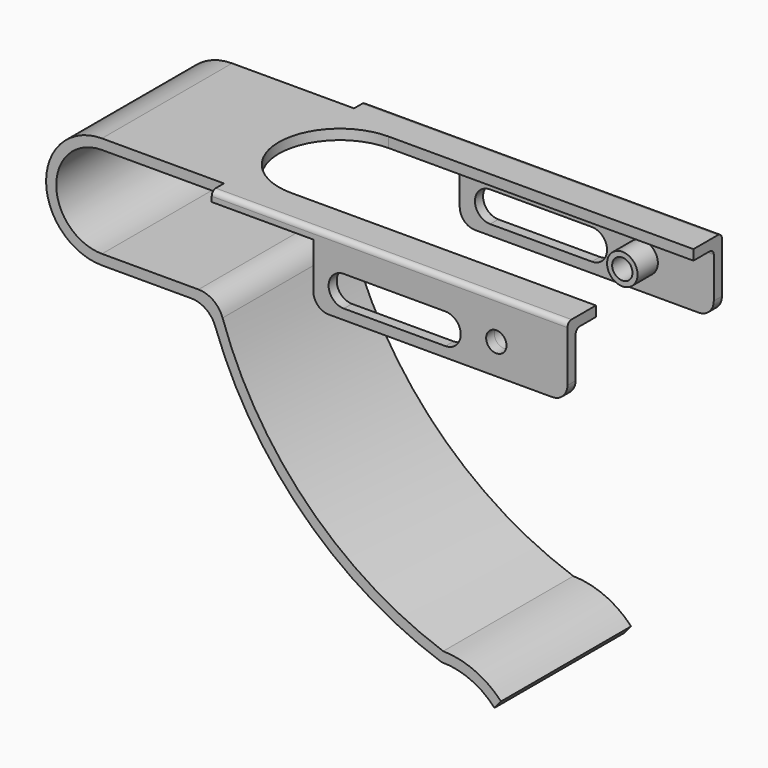
from build123d import *

# Parameters (mm, degrees)
F1_DEPTH  = 16
F2_W      = 70
F2_H      = 3
F3_DEPTH  = 2
F4_W      = 50
F4_H      = 14
F5_DEPTH  = 2
F6_R      = 1
F9_DEPTH  = 2
F11_DEPTH = 38.001
F13_D     = 4
F14_R     = 3
F14_R_2   = 2
F15_DEPTH = 5
F16_R     = 3


# Not quite as in the source:
# - a pattern or mirror of a feature is missing from the dataset's text; its kind, count and spacing are read off the source's solid


with BuildPart() as f1:
    # F0 (on Front) → F1 (new body)
    with BuildSketch(Plane.XZ):
        with BuildLine():
            Line((94, 11), (0, 11))
            ThreePointArc((0, 11), (-11, 0), (0, -11))
            Line((0, -11), (17.5822146692, -11))
            ThreePointArc((17.5822146692, -11), (20.4548889983, -11.9075994576), (22.2846682622, -14.3009031203))
            ThreePointArc((22.2846682622, -14.3009031203), (39.5706846565, -41.223441559), (66.8144425174, -57.9986344457))
            ThreePointArc((66.8144425174, -57.9986344457), (72.5102657096, -59.1645299936), (77.2413235191, -62.5437024171))
            Line((77.2413235191, -62.5437024171), (78.536643648, -61))
            ThreePointArc((78.536643648, -61), (73.3497255449, -57.3487659198), (67.1516242057, -56))
            ThreePointArc((67.1516242057, -56), (40.3930033582, -39.2216179023), (23.7333333333, -12.3889272035))
            ThreePointArc((23.7333333333, -12.3889272035), (21.9107246536, -9.9345748081), (19, -9))
            Line((19, -9), (0, -9))
            ThreePointArc((0, -9), (-9, 0), (0, 9))
            Line((0, 9), (94, 9))
            Line((94, 9), (94, 11))
        make_face()
    extrude(amount=F1_DEPTH)

    # F2 (on face) → F3 (join)
    with BuildSketch(Plane.XY.offset(11)):
        with Locations((59, -17.5)):
            Rectangle(F2_W, F2_H)
    extrude(amount=-F3_DEPTH)

    # F4 (on face) → F5 (join)
    with BuildSketch(Plane.XZ.offset(19)):
        with Locations((69, 4)):
            Rectangle(F4_W, F4_H)
    extrude(amount=-F5_DEPTH)

    # F6
    f6_edges = [f1.edges().sort_by_distance(p)[0] for p in [
        (59, -19, 11),
        (69, -17, 9),
    ]]
    fillet(f6_edges, radius=F6_R)

    # F7: F1 across plane


with BuildPart() as f1_1:
    add(f1.part)
    add(f1.part.mirror(Plane.XZ))

    # F8 (on face) → F9 (cut)
    with BuildSketch(Plane.XY.offset(11)):
        with BuildLine():
            Line((94, 12), (34, 12))
            ThreePointArc((34, 12), (22, 0), (34, -12))
            Line((34, -12), (94, -12))
            Line((94, -12), (94, 12))
        make_face()
    extrude(amount=-F9_DEPTH, mode=Mode.SUBTRACT)

    # F10 (on face) → F11 (cut, through all)
    with BuildSketch(Plane.XZ.offset(19)):
        with BuildLine():
            ThreePointArc((50, 5), (47, 2), (50, -1))
            Line((50, -1), (70, -1))
            ThreePointArc((70, -1), (73, 2), (70, 5))
            Line((70, 5), (50, 5))
        make_face()
    extrude(amount=-F11_DEPTH, mode=Mode.SUBTRACT)

    # F13 (through all)
    with Locations(Plane.XZ.offset(19)):
        with Locations((80, 3)):
            Hole(F13_D / 2)

    # F14 (on face) → F15 (join)
    with BuildSketch(Plane(origin=(0, -17, 0), x_dir=(-1, 0, 0), z_dir=(0, 1, 0))):
        with Locations((-80, 3)):
            Circle(F14_R)
        with Locations((-80, 3)):
            Circle(F14_R_2, mode=Mode.SUBTRACT)
    f15 = extrude(amount=F15_DEPTH)

    # F15_copies: F15 across plane
    add(f15.mirror(Plane.ZX))

    # F16
    f16_edges = [f1_1.edges().sort_by_distance(p)[0] for p in [
        (44, -18, -3),
        (94, -18, -3),
        (44, 18, -3),
        (94, 18, -3),
    ]]
    fillet(f16_edges, radius=F16_R)


solid = f1_1.part
